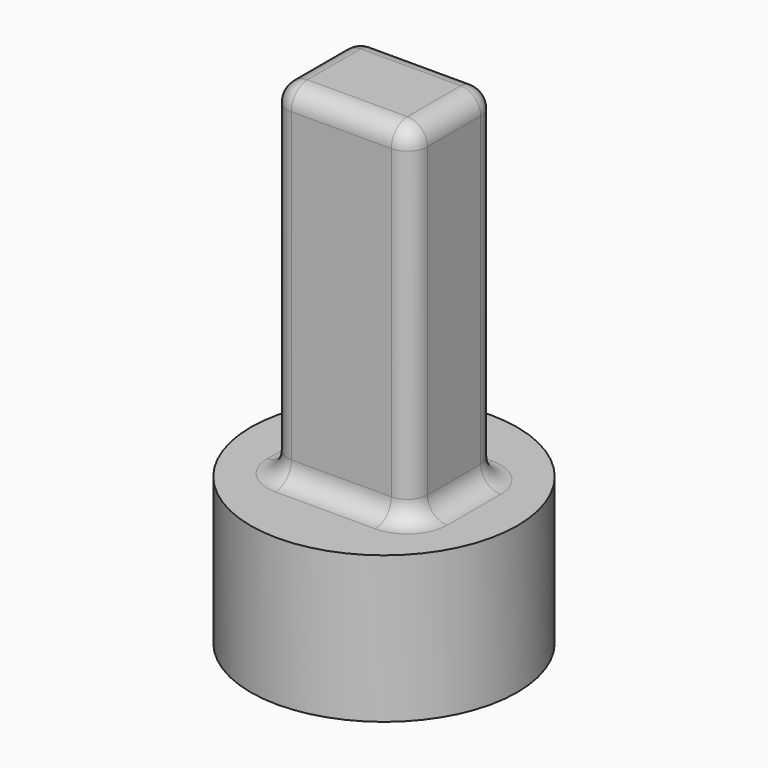
from build123d import *

# Parameters (mm, degrees)
F0_R     = 5
F1_DEPTH = 5.5
F2_W     = 5.25
F2_H     = 4
F3_DEPTH = 13
F4_R     = 0.75
F5_R     = 2.5
F6_DEPTH = 5


with BuildPart() as f1:
    # F0 (on Top) → F1 (new body)
    with BuildSketch(Plane.XY):
        Circle(F0_R)
    extrude(amount=F1_DEPTH)

    # F2 (on face) → F3 (join)
    with BuildSketch(Plane.XY.offset(5.5)):
        Rectangle(F2_W, F2_H)
    extrude(amount=F3_DEPTH)

    # F4
    f4_edges = [f1.edges().sort_by_distance(p)[0] for p in [
        (-2.625, -2, 12),
        (2.625, -2, 12),
        (2.625, 2, 12),
        (-2.625, 2, 12),
        (-2.625, 0, 5.5),
        (-2.625, 0, 18.5),
        (0, -2, 18.5),
        (2.625, 0, 18.5),
        (0, 2, 18.5),
        (0, -2, 5.5),
        (2.625, 0, 5.5),
        (0, 2, 5.5),
    ]]
    fillet(f4_edges, radius=F4_R)

    # F5 (on face) → F6 (cut)
    with BuildSketch(Plane(origin=(0, 0, 0), x_dir=(1, 0, 0), z_dir=(0, 0, -1))):
        Circle(F5_R)
    extrude(amount=-F6_DEPTH, mode=Mode.SUBTRACT)


solid = f1.part
